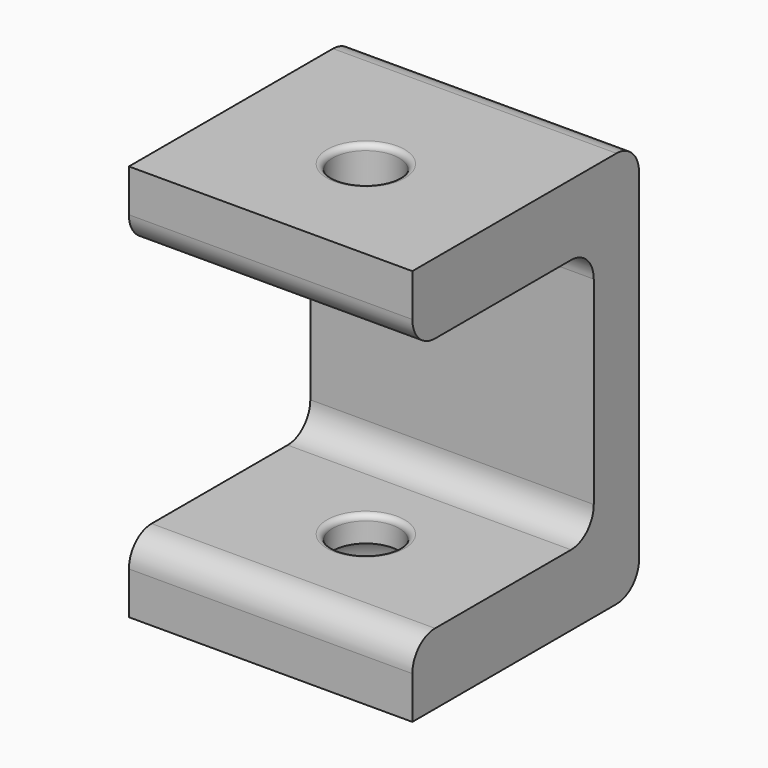
from build123d import *

# Parameters (mm, degrees)
F0_W     = 25
F0_H     = 25
F0_R     = 7
F0_R_2   = 2.925
F1_DEPTH = 35
F2_W     = 25
F2_H     = 22.5
F3_DEPTH = 20
F4_DEPTH = 35.001
F5_R     = 7
F6_DEPTH = 4
F7_R     = 2.5
F8_R     = 3.99999
F9_R     = 0.5


# Not quite as in the source:
# - a fillet or chamfer is up to 0.001 mm smaller than in the source, because OpenCascade refuses the exact size


with BuildPart() as f1:
    # F0 (on Top) → F1 (new body)
    with BuildSketch(Plane.XY):
        Rectangle(F0_W, F0_H)
        with Locations((0, -2)):
            Circle(F0_R, mode=Mode.SUBTRACT)
        with Locations((0, -2)):
            Circle(F0_R)
        with Locations((0, -2)):
            Circle(F0_R_2, mode=Mode.SUBTRACT)
        with Locations((0, -2)):
            Circle(F0_R_2)
    extrude(amount=F1_DEPTH)

    # F2 (on face) → F3 (cut)
    with BuildSketch(Plane.XZ.offset(12.5)):
        with Locations((0, 17.5)):
            Rectangle(F2_W, F2_H)
    extrude(amount=-F3_DEPTH, mode=Mode.SUBTRACT)

    # F0 (on Top) → F4 (cut, through all)
    with BuildSketch(Plane.XY):
        with Locations((0, -2)):
            Circle(F0_R_2)
    extrude(amount=F4_DEPTH, mode=Mode.SUBTRACT)

    # F5 (on face) → F6 (cut)
    with BuildSketch(Plane(origin=(0, 0, 0), x_dir=(1, 0, 0), z_dir=(0, 0, -1))):
        with Locations((0, 2)):
            Circle(F5_R)
    extrude(amount=-F6_DEPTH, mode=Mode.SUBTRACT)

    # F7
    f7_edges = [f1.edges().sort_by_distance(p)[0] for p in [
        (0, 7.5, 6.25),
        (0, 7.5, 28.75),
        (0, 12.5, 35),
        (0, 12.5, 0),
        (0, -12.5, 28.75),
        (0, -12.5, 6.25),
    ]]
    fillet(f7_edges, radius=F7_R)

    # F8 (radius 4 in the source; OpenCascade refuses exactly that, so slightly less here)
    f8_edges = [f1.edges().sort_by_distance(p)[0] for p in [
        (-7, -2, 4),
    ]]
    fillet(f8_edges, radius=F8_R)

    # F9
    f9_edges = [f1.edges().sort_by_distance(p)[0] for p in [
        (-2.925, -2, 35),
        (-2.925, -2, 28.75),
        (-2.925, -2, 6.25),
    ]]
    fillet(f9_edges, radius=F9_R)


solid = f1.part
